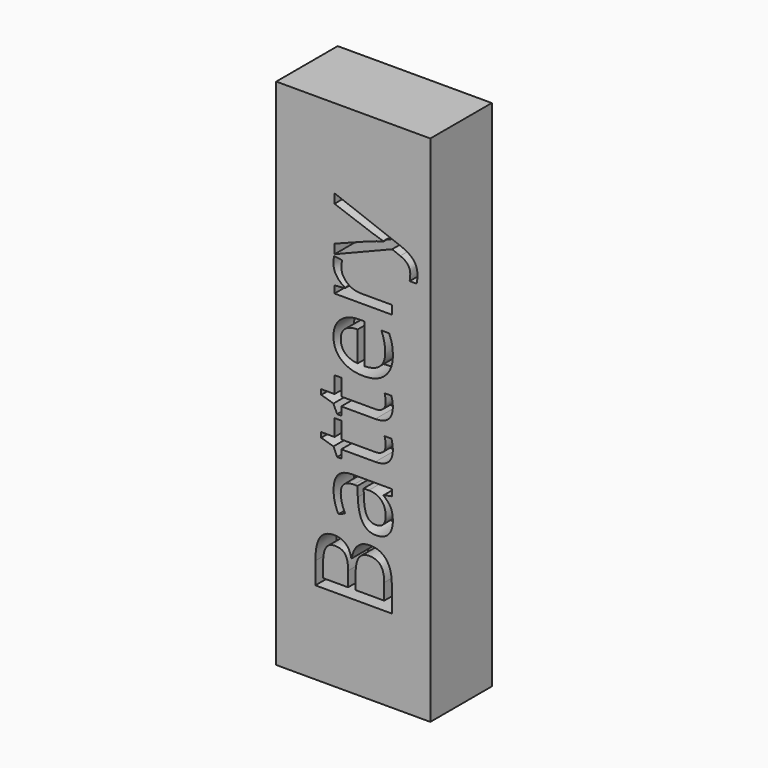
from build123d import *

# Parameters (mm, degrees)
F0_W         = 38.1
F0_H         = 127
F1_DEPTH     = 19
F2_TEXT_SIZE = 26.4583333333
F3_DEPTH     = 6.35


# Not quite as in the source:
# - Text() gives the source's letters only with a copy of the font that has no kerning and outlines rounded to 1/6400 em; it was checked with that copy


with BuildPart() as f1:
    # F0 (on Front) → F1 (new body)
    with BuildSketch(Plane.XZ):
        Rectangle(F0_W, F0_H)
    extrude(amount=F1_DEPTH)

    # F2 (on face) → F3 (cut)
    with BuildSketch(Plane.XZ.offset(19)):
        with Locations(Location((9.525, -45.6034179688), (0, 0, 90))):
            Text('Battery', F2_TEXT_SIZE, font='Open Sans', text_align=(TextAlign.LEFT, TextAlign.BOTTOM))
    extrude(amount=-F3_DEPTH, mode=Mode.SUBTRACT)


solid = f1.part
